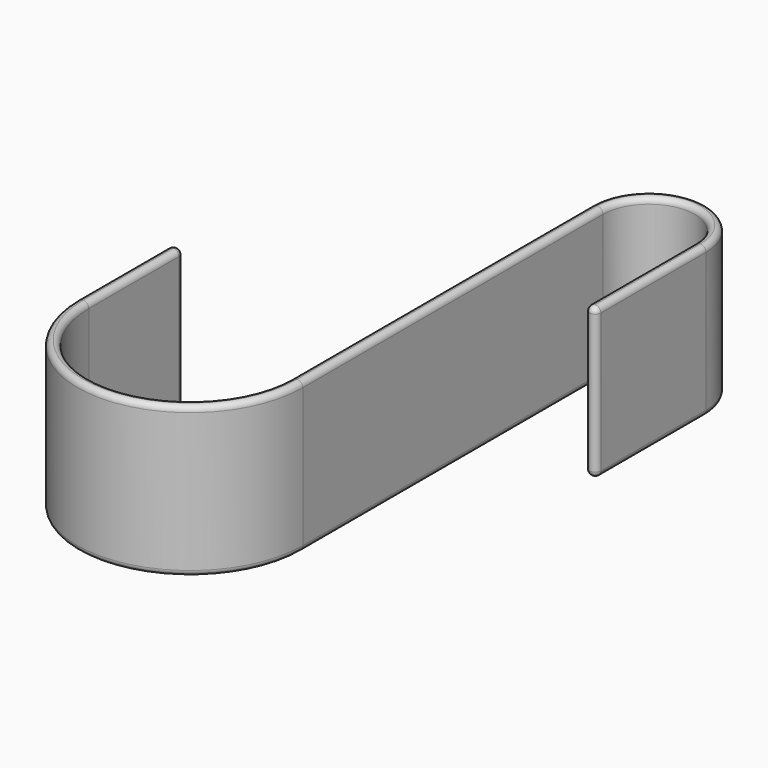
from build123d import *

# Parameters (mm, degrees)
F1_DEPTH = 40
F2_R     = 1.49999


# Not quite as in the source:
# - a fillet or chamfer is up to 0.001 mm smaller than in the source, because OpenCascade refuses the exact size


with BuildPart() as f1:
    # F0 (on Top) → F1 (new body)
    with BuildSketch(Plane.XY):
        with BuildLine():
            ThreePointArc((-30, 0), (0, -30), (30, 0))
            Line((30, 0), (30, 100))
            ThreePointArc((30, 100), (42.1999996752, 112.1999996752), (54.3999993503, 100))
            Line((54.3999993503, 100), (54.3999993503, 65))
            ThreePointArc((54.3999993503, 65), (55.8999993503, 63.5), (57.3999993503, 65))
            Line((57.3999993503, 65), (57.3999993503, 100))
            ThreePointArc((57.3999993503, 100), (42.1999996752, 115.1999996752), (27, 100))
            Line((27, 100), (27, 0))
            ThreePointArc((27, 0), (0, -27), (-27, 0))
            Line((-27, 0), (-27, 30))
            ThreePointArc((-27, 30), (-28.5, 31.5), (-30, 30))
            Line((-30, 30), (-30, 0))
        make_face()
    extrude(amount=F1_DEPTH)

    # F2 (radius 1.5 in the source; OpenCascade refuses exactly that, so slightly less here)
    f2_edges = [f1.edges().sort_by_distance(p)[0] for p in [
        (-30, 15, 40),
        (-30, 15, 0),
    ]]
    fillet(f2_edges, radius=F2_R)


solid = f1.part
